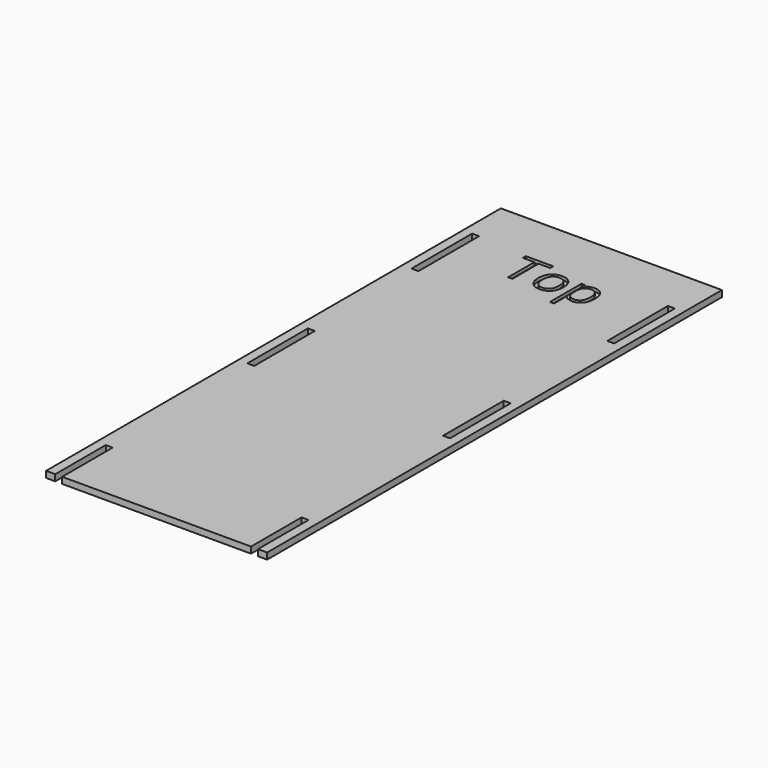
from build123d import *

# Parameters (mm, degrees)
F0_W         = 70
F0_H         = 180
F1_DEPTH     = 2
F2_W         = 2.2
F2_H         = 24
F3_DEPTH     = 25
F4_TEXT_SIZE = 16.1837682956
F5_DEPTH     = 1


# Not quite as in the source:
# - a feature names something its author has since deleted; it is built from what else it names
# - Text() gives the source's letters only with a copy of the font that has no kerning and outlines rounded to 1/6400 em; it was checked with that copy


with BuildPart() as f1:
    # F0 (on Top) → F1 (new body)
    with BuildSketch(Plane.XY):
        with Locations((-0.6928723305, -0.7264627367)):
            Rectangle(F0_W, F0_H)
    extrude(amount=F1_DEPTH)

    # F2 (on Top) → F3 (cut)
    with BuildSketch(Plane.XY):
        with Locations((-31.6928723305, 62.2735372633)):
            Rectangle(F2_W, F2_H)
        with Locations((30.3071276695, 62.2735372633)):
            Rectangle(F2_W, F2_H)
        with Locations((-31.6928723305, -2.7264627367)):
            Rectangle(F2_W, F2_H)
        with Locations((30.3071276695, -2.7264627367)):
            Rectangle(F2_W, F2_H)
        with Locations((-31.6928723305, -82.7264627367)):
            Rectangle(F2_W, F2_H)
        with Locations((30.3071276695, -82.7264627367)):
            Rectangle(F2_W, F2_H)
    extrude(amount=F3_DEPTH, mode=Mode.SUBTRACT)

    # F4 (on face) → F5 (cut)
    with BuildSketch(Plane.XY.offset(2)):
        with Locations((-15.0224762037, 61.5833848715)):
            Text('Top', F4_TEXT_SIZE, font='Open Sans', text_align=(TextAlign.LEFT, TextAlign.BOTTOM))
    extrude(amount=-F5_DEPTH, mode=Mode.SUBTRACT)


solid = f1.part
